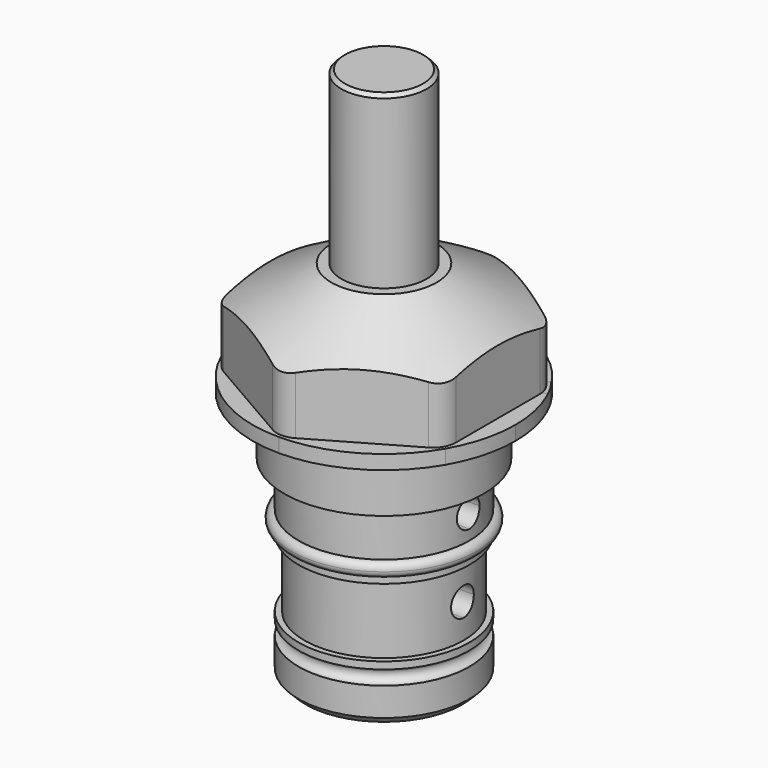
from build123d import *

# Parameters (mm, degrees)
F0_R     = 7.9375
F1_DEPTH = 25.4
F2_DEPTH = 3.175
F3_R     = 5.08
F7_SIZE  = 1.5875
F9_DEPTH = 29.3303937748
F10_W    = 9.525
F10_H    = 47.625
F10_W_2  = 3.175
F10_W_3  = 12.7
F10_H_2  = 12.446
F13_SIZE = 0.79375


with BuildPart() as f1:
    # F0 (on Top) → F1 (new body)
    with BuildSketch(Plane.XY):
        Polygon((25.4, -14.6646968374), (25.4, 14.6646968374), (0, 29.3293936748), (-25.4, 14.6646968374), (-25.4, -14.6646968374), (0, -29.3293936748), align=None)
        Circle(F0_R, mode=Mode.SUBTRACT)
        Circle(F0_R)
    extrude(amount=F1_DEPTH)

    # F0 (on Top) → F2 (join)
    with BuildSketch(Plane.XY):
        with BuildLine():
            ThreePointArc((-25.4, -14.6646968374), (-14.6646968374, -25.4), (0, -29.3293936748))
            Line((0, -29.3293936748), (-25.4, -14.6646968374))
        make_face()
        with BuildLine():
            ThreePointArc((0, -29.3293936748), (14.6646968374, -25.4), (25.4, -14.6646968374))
            Line((25.4, -14.6646968374), (0, -29.3293936748))
        make_face()
        with BuildLine():
            ThreePointArc((25.4, -14.6646968374), (28.3300188199, -7.5910056644), (29.3293936748, 0))
            ThreePointArc((29.3293936748, 0), (28.3300188199, 7.5910056644), (25.4, 14.6646968374))
            Line((25.4, 14.6646968374), (25.4, -14.6646968374))
        make_face()
        Polygon((25.4, -14.6646968374), (25.4, 14.6646968374), (0, 29.3293936748), (-25.4, 14.6646968374), (-25.4, -14.6646968374), (0, -29.3293936748), align=None)
        Circle(F0_R, mode=Mode.SUBTRACT)
        with BuildLine():
            Line((0, 29.3293936748), (25.4, 14.6646968374))
            ThreePointArc((25.4, 14.6646968374), (14.6646968374, 25.4), (0, 29.3293936748))
        make_face()
        with BuildLine():
            Line((-25.4, 14.6646968374), (0, 29.3293936748))
            ThreePointArc((0, 29.3293936748), (-14.6646968374, 25.4), (-25.4, 14.6646968374))
        make_face()
        with BuildLine():
            Line((-25.4, -14.6646968374), (-25.4, 14.6646968374))
            ThreePointArc((-25.4, 14.6646968374), (-29.3293936748, 0), (-25.4, -14.6646968374))
        make_face()
    extrude(amount=F2_DEPTH)

    # F3 (call 1 of 6: OpenCascade refuses the feature's edges together)
    f3_edges = [f1.edges().sort_by_distance(p)[0] for p in [
        (0, -29.329394, 14.2875),
    ]]
    fillet(f3_edges, radius=F3_R)

    # F3#2 (call 2 of 6)
    f3_2_edges = [f1.edges().sort_by_distance(p)[0] for p in [
        (25.4, -14.664697, 14.2875),
    ]]
    fillet(f3_2_edges, radius=F3_R)

    # F3#3 (call 3 of 6)
    f3_3_edges = [f1.edges().sort_by_distance(p)[0] for p in [
        (25.4, 14.664697, 14.2875),
    ]]
    fillet(f3_3_edges, radius=F3_R)

    # F3#4 (call 4 of 6)
    f3_4_edges = [f1.edges().sort_by_distance(p)[0] for p in [
        (0, 29.329394, 14.2875),
    ]]
    fillet(f3_4_edges, radius=F3_R)

    # F3#5 (call 5 of 6)
    f3_5_edges = [f1.edges().sort_by_distance(p)[0] for p in [
        (-25.4, 14.664697, 14.2875),
    ]]
    fillet(f3_5_edges, radius=F3_R)

    # F3#6 (call 6 of 6)
    f3_6_edges = [f1.edges().sort_by_distance(p)[0] for p in [
        (-25.4, -14.664697, 14.2875),
    ]]
    fillet(f3_6_edges, radius=F3_R)

    # F4 (on Right) → F5 (revolve, cut)
    with BuildSketch(Plane.YZ):
        Polygon((35.3962906179, 25.4), (11.7317574699, 25.4), (35.3962906179, 11.7372754168), align=None)
    revolve(axis=Axis((0, 0, 25.9955581278), (0, 0, -1)), mode=Mode.SUBTRACT)

    # F4 (on Right) → F6 (revolve)
    with BuildSketch(Plane.YZ):
        with BuildLine():
            Line((17.78, -27.686), (0, -27.686))
            Line((0, -27.686), (0, -32.131))
            ThreePointArc((0, -32.131), (2.2450640303, -33.0609359697), (3.175, -35.306))
            ThreePointArc((3.175, -35.306), (2.2450640303, -37.5510640303), (0, -38.481))
            Line((0, -38.481), (0, -42.926))
            Line((0, -42.926), (17.78, -42.926))
            Line((17.78, -42.926), (17.78, -27.686))
        make_face()
        with BuildLine():
            Line((19.05, -12.7), (0, -12.7))
            Line((0, -12.7), (0, -14.2875))
            ThreePointArc((0, -14.2875), (2.2450640303, -15.2174359697), (3.175, -17.4625))
            ThreePointArc((3.175, -17.4625), (2.2450640303, -19.7075640303), (0, -20.6375))
            Line((0, -20.6375), (0, -27.686))
            Line((0, -27.686), (17.78, -27.686))
            Line((17.78, -27.686), (19.05, -27.686))
            Line((19.05, -27.686), (19.05, -26.0985))
            ThreePointArc((19.05, -26.0985), (17.4625, -24.511), (19.05, -22.9235))
            Line((19.05, -22.9235), (19.05, -12.7))
        make_face()
        Polygon((22.225, 0), (0, 0), (0, -12.7), (19.05, -12.7), (22.225, -12.7), align=None)
        with BuildLine():
            Line((19.05, -42.926), (17.78, -42.926))
            Line((17.78, -42.926), (0, -42.926))
            Line((0, -42.926), (0, -55.626))
            Line((0, -55.626), (19.05, -55.626))
            Line((19.05, -55.626), (19.05, -47.6885))
            ThreePointArc((19.05, -47.6885), (17.4625, -46.101), (19.05, -44.5135))
            Line((19.05, -44.5135), (19.05, -42.926))
        make_face()
    revolve(axis=Axis((0, 0, 25.9955581278), (0, 0, -1)))

    # F7
    f7_edges = [f1.edges().sort_by_distance(p)[0] for p in [
        (0, -19.05, -55.626),
    ]]
    chamfer(f7_edges, length=F7_SIZE)


with BuildPart() as f8:
    # F4 (on Right) → F8 (revolve)
    with BuildSketch(Plane.YZ):
        with BuildLine():
            Line((0, -20.6375), (0, -14.2875))
            ThreePointArc((0, -14.2875), (-3.175, -17.4625), (0, -20.6375))
        make_face()
    revolve(axis=Axis((0, 0, 25.9955581278), (0, 0, -1)))


with BuildPart() as f8b:
    # F4 (on Right) → F8, piece 2 (revolve)
    with BuildSketch(Plane.YZ):
        with BuildLine():
            ThreePointArc((20.6375, -24.511), (20.1725320151, -23.3884679849), (19.05, -22.9235))
            Line((19.05, -22.9235), (19.05, -26.0985))
            ThreePointArc((19.05, -26.0985), (20.1725320151, -25.6335320151), (20.6375, -24.511))
        make_face()
        with BuildLine():
            Line((19.05, -26.0985), (19.05, -22.9235))
            ThreePointArc((19.05, -22.9235), (17.4625, -24.511), (19.05, -26.0985))
        make_face()
    revolve(axis=Axis((0, 0, 25.9955581278), (0, 0, -1)))


with BuildPart() as f9_tool:
    # F4 (on Right) → F9 (new body, through all)
    with BuildSketch(Plane.YZ):
        with BuildLine():
            Line((0, -20.6375), (0, -14.2875))
            ThreePointArc((0, -14.2875), (-3.175, -17.4625), (0, -20.6375))
        make_face()
        with BuildLine():
            ThreePointArc((3.175, -17.4625), (2.2450640303, -15.2174359697), (0, -14.2875))
            Line((0, -14.2875), (0, -20.6375))
            ThreePointArc((0, -20.6375), (2.2450640303, -19.7075640303), (3.175, -17.4625))
        make_face()
        with BuildLine():
            Line((0, -38.481), (0, -32.131))
            ThreePointArc((0, -32.131), (-3.175, -35.306), (0, -38.481))
        make_face()
        with BuildLine():
            ThreePointArc((3.175, -35.306), (2.2450640303, -33.0609359697), (0, -32.131))
            Line((0, -32.131), (0, -38.481))
            ThreePointArc((0, -38.481), (2.2450640303, -37.5510640303), (3.175, -35.306))
        make_face()
    extrude(amount=F9_DEPTH)


with BuildPart() as f1_1:
    add(f1.part)

    # F9: cut by f9_tool
    add(f9_tool.part, mode=Mode.SUBTRACT)


with BuildPart() as f8_1:
    add(f8.part)

    # F9: cut by f9_tool
    add(f9_tool.part, mode=Mode.SUBTRACT)


with BuildPart() as f11_tool:
    # F10 (on Right) → F11 (revolve)
    with BuildSketch(Plane.YZ):
        Polygon((9.525, 63.5), (0, 63.5), (0, 15.875), (9.525, 15.875), (9.525, 21.374261314), align=None)
        Polygon((9.525, 21.374261314), (9.525, 15.875), (12.7, 15.875), align=None)
        with Locations((4.7625, -7.9375)):
            Rectangle(F10_W, F10_H)
        with Locations((11.1125, -7.9375)):
            Rectangle(F10_W_2, F10_H)
        with Locations((6.35, -44.323)):
            Rectangle(F10_W_3, F10_H_2)
        Polygon((9.525, -31.75), (0, -31.75), (0, -38.1), (12.7, -38.1), (12.7, -31.75), align=None)
    revolve(axis=Axis((0, 0, 6.477), (0, 0, -1)))


with BuildPart() as f1_2:
    add(f1_1.part)

    # F11: cut by f11_tool
    add(f11_tool.part, mode=Mode.SUBTRACT)


with BuildPart() as f8_2:
    add(f8_1.part)

    # F11: cut by f11_tool
    add(f11_tool.part, mode=Mode.SUBTRACT)


with BuildPart() as f12:
    # F10 (on Right) → F12 (revolve)
    with BuildSketch(Plane.YZ):
        Polygon((9.525, 63.5), (0, 63.5), (0, 15.875), (9.525, 15.875), (9.525, 21.374261314), align=None)
        with Locations((4.7625, -7.9375)):
            Rectangle(F10_W, F10_H)
        Polygon((9.525, -31.75), (0, -31.75), (0, -38.1), (12.7, -38.1), (12.7, -31.75), align=None)
    revolve(axis=Axis((0, 0, 6.477), (0, 0, -1)))

    # F13
    f13_edges = [f12.edges().sort_by_distance(p)[0] for p in [
        (0, -9.525, 63.5),
    ]]
    chamfer(f13_edges, length=F13_SIZE)


solid = Compound([f8b.part, f1_2.part, f12.part])
